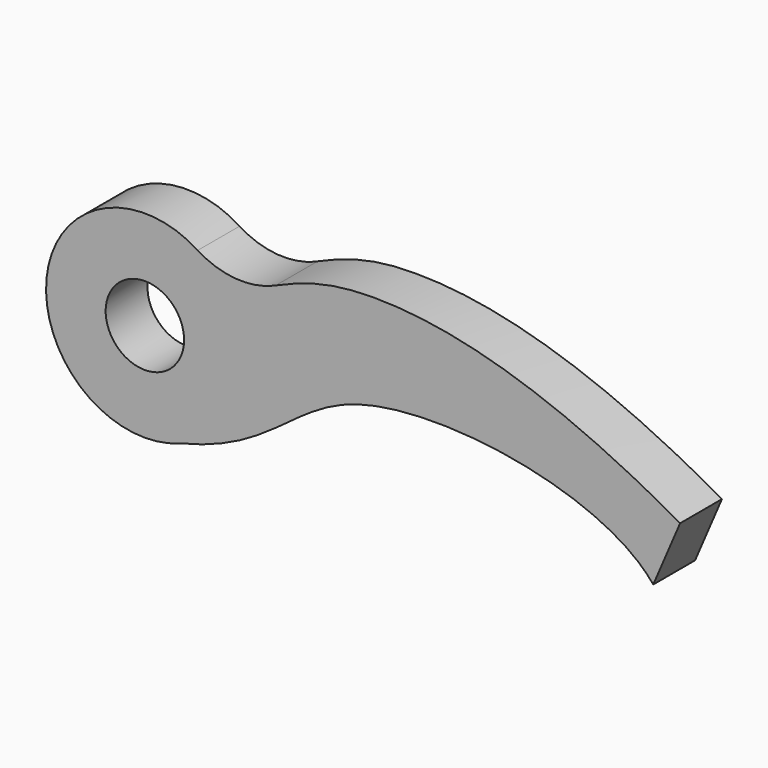
from build123d import *

# Parameters (mm, degrees)
F1_DEPTH = 3.175
F2_R     = 5


# Not quite as in the source:
# - a length typed as a fraction of an inch, garbled in the dataset ("3 / 203.2 mm" for 3/8 in), is restored


with BuildPart() as f1:
    # F0 (on Front) → F1 (new body)
    with BuildSketch(Plane.XZ):
        with BuildLine():
            ThreePointArc((6, 0), (5.7619448426, 1.6733175524), (5.0666694563, 3.2138544803))
            ThreePointArc((5.0666694563, 3.2138544803), (0.0307741544, 5.9999210788), (-5.0334354285, 3.2656588595))
            ThreePointArc((-5.0334354285, 3.2656588595), (-5.2722838105, -2.8640920763), (0, -6))
            add(Edge.make_bspline(
                [(0, -6), (0.7881316779, -5.8923160671), (1.5037462454, -5.7565864603), (2.1584342276, -5.5983177549)],
                knots=[0, 0, 0, 0, 0.0486422356, 0.0486422356, 0.0486422356, 0.0486422356], degree=3))
            ThreePointArc((2.1584342276, -5.5983177549), (3.7803533787, -4.6592841008), (5.0334354285, -3.2656588595))
            ThreePointArc((5.0334354285, -3.2656588595), (5.7532865638, -1.7028487057), (6, 0))
        make_face()
        with BuildLine():
            ThreePointArc((1.9898590203, 1.3079803675), (2.281304819, 0.6826418425), (2.38125, 0))
            ThreePointArc((2.38125, 0), (-2.281304819, -0.6826418425), (1.9898590203, 1.3079803675))
        make_face(mode=Mode.SUBTRACT)
        with BuildLine():
            add(Edge.make_bspline(
                [(5.0666694563, 3.2138544803), (8.837595406, 5.414485816), (14.2440437805, 6.8995614863), (24.1781340673, 4.7387528577), (32.5091555715, 0)],
                knots=[0.1268767178, 0.1268767178, 0.1268767178, 0.1268767178, 0.46554979, 1, 1, 1, 1], degree=3))
            ThreePointArc((5.0666694563, 3.2138544803), (5.7619448426, 1.6733175524), (6, 0))
            ThreePointArc((6, 0), (5.7532865638, -1.7028487057), (5.0334354285, -3.2656588595))
            ThreePointArc((5.0334354285, -3.2656588595), (3.7803533787, -4.6592841008), (2.1584342276, -5.5983177549))
            add(Edge.make_bspline(
                [(2.1584342276, -5.5983177549), (7.8149044031, -4.2308843573), (10.3239452596, 2.6732879939), (27.8337137958, 0), (30.8784303042, -3.806720163)],
                knots=[0.0486422356, 0.0486422356, 0.0486422356, 0.0486422356, 0.4689086255, 1, 1, 1, 1], degree=3))
            Line((30.8784303042, -3.806720163), (32.5091555715, 0))
        make_face()
        with BuildLine():
            add(Edge.make_bspline(
                [(0, -6), (0.7881316779, -5.8923160671), (1.5037462454, -5.7565864603), (2.1584342276, -5.5983177549)],
                knots=[0, 0, 0, 0, 0.0486422356, 0.0486422356, 0.0486422356, 0.0486422356], degree=3))
            ThreePointArc((0, -6), (1.0977462071, -5.8987247151), (2.1584342276, -5.5983177549))
        make_face()
    extrude(amount=F1_DEPTH)

    # F2
    f2_edges = [f1.edges().sort_by_distance(p)[0] for p in [
        (5.066669, -1.5875, 3.213854),
    ]]
    fillet(f2_edges, radius=F2_R)


solid = f1.part
